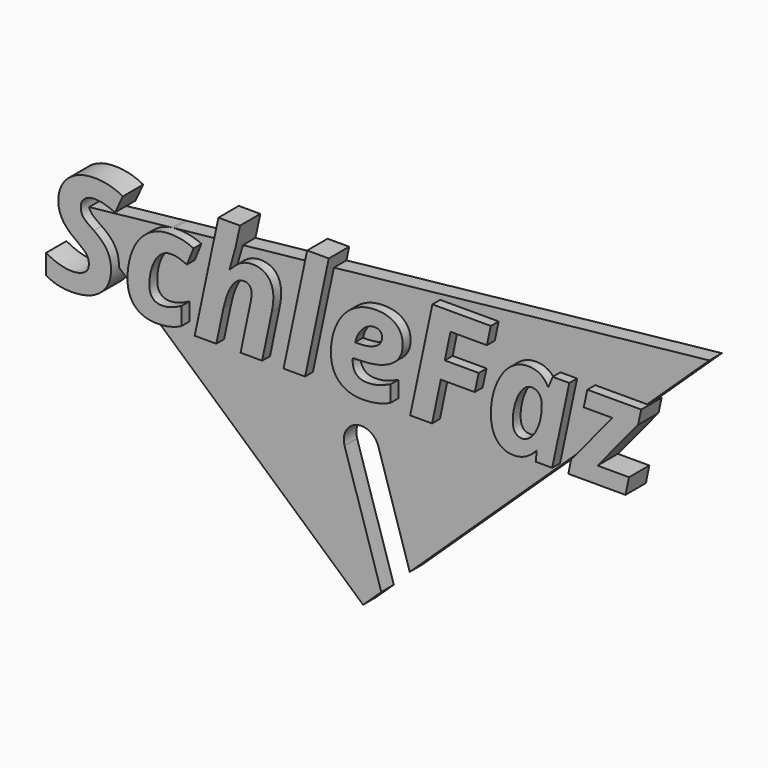
from build123d import *

# Parameters (mm, degrees)
F1_DEPTH     = 1.6
F2_TEXT_SIZE = 15.0013232014
F3_DEPTH     = 2.6
F5_DEPTH     = 12.5


# Not quite as in the source:
# - Text() gives the source's letters only with a copy of the font that has no kerning and outlines rounded to 1/6400 em; it was checked with that copy


with BuildPart() as f1:
    # F0 (on Front) → F1 (new body)
    with BuildSketch(Plane.XZ):
        Polygon((39.5777293295, 8.3956420519), (-25.4222706705, 1.4043629969), (4.2434261745, -25.0491239228), align=None)
    extrude(amount=F1_DEPTH)

    # F2 (on Front) → F3 (join)
    with BuildSketch(Plane.XZ):
        with Locations((-27.606235873, -5.8049081583)):
            Text('SchleFaz', F2_TEXT_SIZE, font='Open Sans', font_style=FontStyle.BOLDITALIC, text_align=(TextAlign.LEFT, TextAlign.BOTTOM))
    extrude(amount=F3_DEPTH)

    # F4 (on Front) → F5 (cut, symmetric)
    with BuildSketch(Plane.XZ):
        with BuildLine():
            Line((2.3546157788, -11.3750521068), (6.3059052648, -23.9697855854))
            Line((6.3059052648, -23.9697855854), (9.7408325771, -22.8921611802))
            Line((9.7408325771, -22.8921611802), (5.7895430912, -10.2974277015))
            ThreePointArc((5.7895430912, -10.2974277015), (3.5332672324, -9.118776248), (2.3546157788, -11.3750521068))
        make_face()
    extrude(amount=F5_DEPTH, both=True, mode=Mode.SUBTRACT)


solid = f1.part
